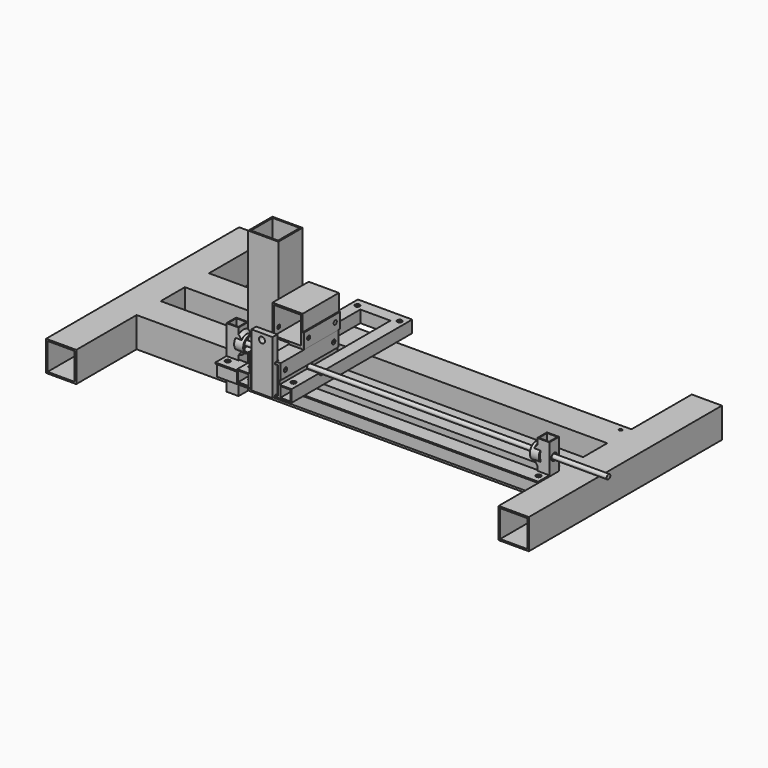
from build123d import *

# Parameters (mm, degrees)
F0_W           = 50
F0_H           = 50
F0_W_2         = 45
F0_H_2         = 45
F1_DEPTH       = 200
F2_W           = 50
F2_H           = 50
F2_W_2         = 45
F2_H_2         = 45
F3_DEPTH       = 700
F4_W           = 20
F4_H           = 20
F4_W_2         = 17
F4_H_2         = 17
F5_DEPTH       = 50
F6_DEPTH       = 50
F7_W           = 20
F7_H           = 20
F7_W_2         = 17
F7_H_2         = 17
F8_DEPTH       = 535
F9_R           = 6
F10_DEPTH      = 750.001
F11_R          = 13
F11_R_2        = 11
F12_DEPTH      = 10
F13_DEPTH      = 5
F14_R          = 13
F14_R_2        = 11
F15_DEPTH      = 10
F16_DEPTH      = 5
F17_T4_ANGLE   = 213.9701071651
F17_T10_ANGLE  = 213.9701071651
F17_T16_ANGLE  = 213.9701071651
F17_T22_ANGLE  = 213.9701071651
F18_R          = 2.5
F19_DEPTH      = 10
F21_DEPTH      = 535
F22_W          = 20
F22_H          = 2
F22_R          = 4
F23_DEPTH      = 26
F24_R          = 3.8004541597
F25_DEPTH      = 535
F25_DEPTH_BACK = 90
F27_DEPTH      = 64
F28_R          = 3.25
F29_DEPTH      = 60.5
F30_W          = 20
F30_H          = 20
F30_W_2        = 17
F30_H_2        = 17
F30_W_3        = 45
F30_H_3        = 45
F31_DEPTH      = 90
F31_DEPTH_BACK = 30
F32_R          = 6
F32_R_2        = 3.25
F33_DEPTH      = 100.4
F34_W          = 20
F34_H          = 20
F34_W_2        = 17
F34_H_2        = 17
F35_DEPTH      = 130
F37_W          = 20
F37_H          = 20
F37_W_2        = 17
F37_H_2        = 17
F38_DEPTH      = 50
F36_W          = 35
F36_H          = 5
F36_R          = 4
F39_DEPTH      = 87
F40_W          = 50
F40_H          = 50
F40_W_2        = 45
F40_H_2        = 45
F41_DEPTH      = 200
F44_DEPTH      = 120
F45_W          = 17.5
F45_H          = 5
F46_DEPTH      = 34
F47_W          = 35
F47_H          = 89
F47_R          = 5
F48_DEPTH      = 10
F49_W          = 50
F49_H          = 50
F49_W_2        = 45
F49_H_2        = 45
F50_DEPTH      = 75
F51_R          = 3.5312662509
F52_DEPTH      = 25
F53_R          = 3
F54_DEPTH      = 106.1
F56_DEPTH      = 75
F57_R          = 3.25
F58_DEPTH      = 25


# Not quite as in the source:
# - a fillet or chamfer that OpenCascade refuses, or shapes differently, is made with other operations: its cross-section is extruded or revolved along the edge and cut away or added


with BuildPart() as f1:
    # F0 (on Front) → F1 (new body, symmetric)
    with BuildSketch(Plane.XZ):
        with Locations((-375, 0)):
            Rectangle(F0_W, F0_H)
        with Locations((-375, 0)):
            Rectangle(F0_W_2, F0_H_2, mode=Mode.SUBTRACT)
    extrude(amount=F1_DEPTH, both=True)



with BuildPart() as f1b:
    # F0 (on Front) → F1, piece 2 (new body, symmetric)
    with BuildSketch(Plane.XZ):
        with Locations((375, 0)):
            Rectangle(F0_W, F0_H)
        with Locations((375, 0)):
            Rectangle(F0_W_2, F0_H_2, mode=Mode.SUBTRACT)
    extrude(amount=F1_DEPTH, both=True)


with BuildPart() as f1_1:
    add(f1.part)

    add(f1b.part)  # F3 merges F1b
    # F2 (on face) → F3 (join, through all)
    with BuildSketch(Plane.YZ.offset(-350)):
        with Locations((50, 0)):
            Rectangle(F2_W, F2_H)
        with Locations((50, 0)):
            Rectangle(F2_W_2, F2_H_2, mode=Mode.SUBTRACT)
        with Locations((-50, 0)):
            Rectangle(F2_W, F2_H)
        with Locations((-50, 0)):
            Rectangle(F2_W_2, F2_H_2, mode=Mode.SUBTRACT)
    extrude(amount=F3_DEPTH)

    # F4 (on face) → F5 (join)
    with BuildSketch(Plane.XY.offset(25)):
        with Locations((340, -85)):
            Rectangle(F4_W, F4_H)
        with Locations((340, -85)):
            Rectangle(F4_W_2, F4_H_2, mode=Mode.SUBTRACT)
        with Locations((-175, -85)):
            Rectangle(F4_W, F4_H)
        with Locations((-175, -85)):
            Rectangle(F4_W_2, F4_H_2, mode=Mode.SUBTRACT)
    extrude(amount=-F5_DEPTH)

    # F4 (on face) → F6 (join)
    with BuildSketch(Plane.XY.offset(25)):
        with Locations((340, -85)):
            Rectangle(F4_W, F4_H)
        with Locations((340, -85)):
            Rectangle(F4_W_2, F4_H_2, mode=Mode.SUBTRACT)
        with Locations((-175, -85)):
            Rectangle(F4_W, F4_H)
        with Locations((-175, -85)):
            Rectangle(F4_W_2, F4_H_2, mode=Mode.SUBTRACT)
    extrude(amount=F6_DEPTH)

    # F7 (on face) → F8 (join)
    with BuildSketch(Plane(origin=(350, 0, 0), x_dir=(0, -1, 0), z_dir=(-1, 0, 0))):
        with Locations((105, 15)):
            Rectangle(F7_W, F7_H)
        with Locations((105, 15)):
            Rectangle(F7_W_2, F7_H_2, mode=Mode.SUBTRACT)
    extrude(amount=F8_DEPTH)

    # F9 (on face) → F10 (cut, through all)
    with BuildSketch(Plane.YZ.offset(350)):
        with Locations((-85, 50)):
            Circle(F9_R)
    extrude(amount=-F10_DEPTH, mode=Mode.SUBTRACT)

    # F11 (on face) → F12 (join)
    with BuildSketch(Plane(origin=(330, 0, 0), x_dir=(0, -1, 0), z_dir=(-1, 0, 0))):
        with Locations((85, 50)):
            Circle(F11_R)
        with Locations((85, 50)):
            Circle(F11_R_2, mode=Mode.SUBTRACT)
    extrude(amount=F12_DEPTH)

    # F11 (on face) → F13 (join)
    with BuildSketch(Plane(origin=(330, 0, 0), x_dir=(0, -1, 0), z_dir=(-1, 0, 0))):
        with Locations((85, 50)):
            Circle(F11_R)
        with Locations((85, 50)):
            Circle(F11_R_2, mode=Mode.SUBTRACT)
    extrude(amount=-F13_DEPTH)

    # F14 (on face) → F15 (join)
    with BuildSketch(Plane.YZ.offset(-165)):
        with Locations((-85, 50)):
            Circle(F14_R)
        with Locations((-85, 50)):
            Circle(F14_R_2, mode=Mode.SUBTRACT)
    extrude(amount=F15_DEPTH)

    # F14 (on face) → F16 (join)
    with BuildSketch(Plane.YZ.offset(-165)):
        with Locations((-85, 50)):
            Circle(F14_R)
        with Locations((-85, 50)):
            Circle(F14_R_2, mode=Mode.SUBTRACT)
    extrude(amount=-F16_DEPTH)

    # F17: chamfer of 5 on 10 edges, made by hand


with BuildPart() as f17_tool2:
    # F17_s3 → F17_t4 (revolve)
    with BuildSketch(Plane(origin=(0, 6.7154986509, 21.9859176279), x_dir=(1, 0, 0), z_dir=(0, 0.2921222291, 0.9563809927))):
        Polygon((-165, -113.8984958377), (-160, -108.8984958377), (-165, -108.8984958377), align=None)
    revolve(axis=Axis((-165, -85, 50), (1, 0, 0)), revolution_arc=F17_T4_ANGLE)

    split(bisect_by=Plane.XZ.offset(75), keep=Keep.TOP)

    split(bisect_by=Plane.XZ.offset(95), keep=Keep.BOTTOM)


with BuildPart() as f1_2:
    add(f1_1.part)

    # F17_t1: union F17_tool2
    add(f17_tool2.part)


with BuildPart() as f17_tool8:
    # F17_s9 → F17_t10 (revolve)
    with BuildSketch(Plane(origin=(0, 6.7154986509, 21.9859176279), x_dir=(1, 0, 0), z_dir=(0, -0.2921222291, -0.9563809927))):
        Polygon((-165, 77.8984958377), (-160, 82.8984958377), (-165, 82.8984958377), align=None)
    revolve(axis=Axis((-165, -85, 50), (1, 0, 0)), revolution_arc=F17_T10_ANGLE)

    split(bisect_by=Plane.XZ.offset(75), keep=Keep.TOP)

    split(bisect_by=Plane.XZ.offset(95), keep=Keep.BOTTOM)


with BuildPart() as f1_3:
    add(f1_2.part)

    # F17_t7: union F17_tool8
    add(f17_tool8.part)


with BuildPart() as f17_tool14:
    # F17_s15 → F17_t16 (revolve)
    with BuildSketch(Plane(origin=(0, -21.2225160964, 69.4805426982), x_dir=(1, 0, 0), z_dir=(0, -0.2921222291, 0.9563809927))):
        Polygon((330, -48.686272927), (325, -53.686272927), (330, -53.686272927), align=None)
    revolve(axis=Axis((330, -85, 50), (-1, 0, 0)), revolution_arc=F17_T16_ANGLE)

    split(bisect_by=Plane.XZ.offset(75), keep=Keep.TOP)

    split(bisect_by=Plane.XZ.offset(95), keep=Keep.BOTTOM)


with BuildPart() as f1_4:
    add(f1_3.part)

    # F17_t13: union F17_tool14
    add(f17_tool14.part)


with BuildPart() as f17_tool20:
    # F17_s21 → F17_t22 (revolve)
    with BuildSketch(Plane(origin=(0, -21.2225160964, 69.4805426982), x_dir=(1, 0, 0), z_dir=(0, 0.2921222291, -0.9563809927))):
        Polygon((330, 84.686272927), (325, 79.686272927), (330, 79.686272927), align=None)
    revolve(axis=Axis((330, -85, 50), (-1, 0, 0)), revolution_arc=F17_T22_ANGLE)

    split(bisect_by=Plane.XZ.offset(75), keep=Keep.TOP)

    split(bisect_by=Plane.XZ.offset(95), keep=Keep.BOTTOM)


with BuildPart() as f1_5:
    add(f1_4.part)

    # F17_t19: union F17_tool20
    add(f17_tool20.part)

    # F18 (on face) → F19 (cut)
    with BuildSketch(Plane.XY.offset(25)):
        with Locations((-175, -65)):
            Circle(F18_R)
        with Locations((-175, 65)):
            Circle(F18_R)
        with Locations((-175, -105)):
            Circle(F18_R)
        with Locations((340, -105)):
            Circle(F18_R)
        with Locations((340, -65)):
            Circle(F18_R)
        with Locations((340, 65)):
            Circle(F18_R)
    extrude(amount=-F19_DEPTH, mode=Mode.SUBTRACT)

    # F40 (on face) → F41 (join)
    with BuildSketch(Plane(origin=(0, 0, -25), x_dir=(1, 0, 0), z_dir=(0, 0, -1))):
        with Locations((-180, 0)):
            Rectangle(F40_W, F40_H)
        with Locations((-180, 0)):
            Rectangle(F40_W_2, F40_H_2, mode=Mode.SUBTRACT)
    extrude(amount=-F41_DEPTH)


with BuildPart() as f21:
    # F20 (on face) → F21 (new body)
    with BuildSketch(Plane.YZ.offset(350)):
        Polygon((-118, 27), (-118, 25), (-95, 25), (-95, 2), (-93, 2), (-93, 27), align=None)
    extrude(amount=-F21_DEPTH)

    # F22 (on face) → F23 (cut)
    with BuildSketch(Plane.XY.offset(27)):
        with Locations((-175, -94)):
            Rectangle(F22_W, F22_H)
        with Locations((340, -94)):
            Rectangle(F22_W, F22_H)
        with Locations((-175, -105)):
            Circle(F22_R)
        with Locations((340, -105)):
            Circle(F22_R)
    extrude(amount=-F23_DEPTH, mode=Mode.SUBTRACT)


with BuildPart() as f25:
    # F24 (on face) → F25 (new body, two sides)
    with BuildSketch(Plane.YZ.offset(350)) as f25_sk:
        with Locations((-85, 50)):
            Circle(F24_R)
    extrude(amount=-F25_DEPTH)
    extrude(f25_sk.sketch, amount=F25_DEPTH_BACK)


with BuildPart() as f27:
    # F26 (on face) → F27 (new body)
    with BuildSketch(Plane.XZ.offset(118)):
        Polygon((-126.8333580792, 52), (-126.8333580792, 27), (-101.8333580792, 27), (-101.8333580792, 29), (-124.8333580792, 29), (-124.8333580792, 52), align=None)
    extrude(amount=-F27_DEPTH)

    # F28 (on face) → F29 (cut)
    with BuildSketch(Plane(origin=(-126.8333580792, 0, 0), x_dir=(0, -1, 0), z_dir=(-1, 0, 0))):
        with BuildLine():
            Line((79, 58), (79, 50))
            ThreePointArc((79, 50), (85, 44), (91, 50))
            Line((91, 50), (91, 58))
            Line((91, 58), (79, 58))
        make_face()
        with Locations((64, 39)):
            Circle(F28_R)
        with Locations((108, 39)):
            Circle(F28_R)
    extrude(amount=-F29_DEPTH, mode=Mode.SUBTRACT)


with BuildPart() as f31:
    # F30 (on face) → F31 (new body, two sides)
    with BuildSketch(Plane.XZ.offset(118)) as f31_sk:
        with Locations((-114.8333580792, 39)):
            Rectangle(F30_W, F30_H)
        with Locations((-114.8333580792, 39)):
            Rectangle(F30_W_2, F30_H_2, mode=Mode.SUBTRACT)
        Polygon((-104.8333580792, 49), (-104.8333580792, 29), (-54.8333580792, 29), (-54.8333580792, 49), (-54.8333580792, 79), (-104.8333580792, 79), align=None)
        with Locations((-79.8333580792, 54)):
            Rectangle(F30_W_3, F30_H_3, mode=Mode.SUBTRACT)
        with Locations((-44.8333580792, 39)):
            Rectangle(F30_W, F30_H)
        with Locations((-44.8333580792, 39)):
            Rectangle(F30_W_2, F30_H_2, mode=Mode.SUBTRACT)
    extrude(amount=-F31_DEPTH)
    extrude(f31_sk.sketch, amount=F31_DEPTH_BACK)

    # F32 (on face) → F33 (cut)
    with BuildSketch(Plane.YZ.offset(-34.8333580792)):
        with Locations((-85, 50)):
            Circle(F32_R)
        with Locations((-138, 67.5)):
            Circle(F32_R_2)
        with Locations((-38, 67.5)):
            Circle(F32_R_2)
    extrude(amount=-F33_DEPTH, mode=Mode.SUBTRACT)

    # F34 (on face) → F35 (join)
    with BuildSketch(Plane(origin=(0, -28, 0), x_dir=(-1, 0, 0), z_dir=(0, 1, 0))):
        with Locations((44.8333580792, 39)):
            Rectangle(F34_W, F34_H)
        with Locations((44.8333580792, 39)):
            Rectangle(F34_W_2, F34_H_2, mode=Mode.SUBTRACT)
        with Locations((114.8333580792, 39)):
            Rectangle(F34_W, F34_H)
        with Locations((114.8333580792, 39)):
            Rectangle(F34_W_2, F34_H_2, mode=Mode.SUBTRACT)
    extrude(amount=F35_DEPTH)

    # F37 (on face) → F38 (join, through all)
    with BuildSketch(Plane.YZ.offset(-104.8333580792)):
        with Locations((92, 39)):
            Rectangle(F37_W, F37_H)
        with Locations((92, 39)):
            Rectangle(F37_W_2, F37_H_2, mode=Mode.SUBTRACT)
    extrude(amount=F38_DEPTH)

    # F36 (on face) → F39 (cut)
    with BuildSketch(Plane.XY.offset(79)):
        with Locations((-79.8333580792, -145.5)):
            Rectangle(F36_W, F36_H)
        with Locations((-114.8333580792, -131.5)):
            Circle(F36_R)
        with Locations((-44.8333580792, -131.5)):
            Circle(F36_R)
        with Locations((-44.8333580792, 88.5)):
            Circle(F36_R)
        with Locations((-114.8333580792, 88.5)):
            Circle(F36_R)
        with Locations((-79.8333580792, -30.5)):
            Rectangle(F36_W, F36_H)
    extrude(amount=-F39_DEPTH, mode=Mode.SUBTRACT)

    # F47 (on face) → F48 (join)
    with BuildSketch(Plane.XZ.offset(143)):
        with Locations((-79.8333580792, 73.5)):
            Rectangle(F47_W, F47_H)
        with Locations((-79.8333580792, 108)):
            Circle(F47_R, mode=Mode.SUBTRACT)
    extrude(amount=F48_DEPTH)


with BuildPart() as f44:
    # F43 (on face) → F44 (new body)
    with BuildSketch(Plane.XZ.offset(148)):
        Polygon((-77.8333580792, 79), (-54.8333580792, 79), (-54.8333580792, 56), (-52.8333580792, 56), (-52.8333580792, 81), (-77.8333580792, 81), align=None)
    extrude(amount=-F44_DEPTH)

    # F45 (on face) → F46 (cut)
    with BuildSketch(Plane.XY.offset(81)):
        with Locations((-69.0833580792, -145.5)):
            Rectangle(F45_W, F45_H)
        with Locations((-69.0833580792, -30.5)):
            Rectangle(F45_W, F45_H)
    extrude(amount=-F46_DEPTH, mode=Mode.SUBTRACT)

    # F42 (on face) + F51 (on face) → F52 (cut)
    with BuildSketch(Plane.YZ.offset(-155)):
        with BuildLine():
            ThreePointArc((25, 97.8345367185), (45.1040463817, 117.1322684247), (52.5, 144))
            ThreePointArc((52.5, 144), (-26.8677315753, 189.1040463817), (-25, 97.8345367185))
            Line((-25, 97.8345367185), (-25, 175))
            Line((-25, 175), (25, 175))
            Line((25, 175), (25, 97.8345367185))
        make_face()
    with BuildSketch(Plane.YZ.offset(-52.8333580792)):
        with Locations((-138, 67.5)):
            Circle(F51_R)
        with Locations((-38, 67.5)):
            Circle(F51_R)
    extrude(amount=-F52_DEPTH, mode=Mode.SUBTRACT)


with BuildPart() as f50:
    # F49 (on face) → F50 (new body)
    with BuildSketch(Plane.XZ.offset(25)):
        with Locations((-79.8333580792, 108)):
            Rectangle(F49_W, F49_H)
        with Locations((-79.8333580792, 108)):
            Rectangle(F49_W_2, F49_H_2, mode=Mode.SUBTRACT)
    extrude(amount=F50_DEPTH)

    # F53 (on face) → F54 (cut)
    with BuildSketch(Plane.YZ.offset(-54.8333580792)):
        with Locations((-90, 94.5)):
            Circle(F53_R)
        with Locations((-35, 94.5)):
            Circle(F53_R)
    extrude(amount=-F54_DEPTH, mode=Mode.SUBTRACT)


with BuildPart() as f56:
    # F55 (on face) → F56 (new body)
    with BuildSketch(Plane.XZ.offset(100)):
        Polygon((-54.8333580792, 83), (-77.8333580792, 83), (-77.8333580792, 81), (-52.8333580792, 81), (-52.8333580792, 106), (-54.8333580792, 106), align=None)
    extrude(amount=-F56_DEPTH)

    # F57 (on face) → F58 (cut)
    with BuildSketch(Plane.YZ.offset(-52.8333580792)):
        with Locations((-90, 94.5)):
            Circle(F57_R)
        with Locations((-35, 94.5)):
            Circle(F57_R)
    extrude(amount=-F58_DEPTH, mode=Mode.SUBTRACT)


solid = Compound([f1_5.part, f21.part, f25.part, f27.part, f31.part, f44.part, f50.part, f56.part])
